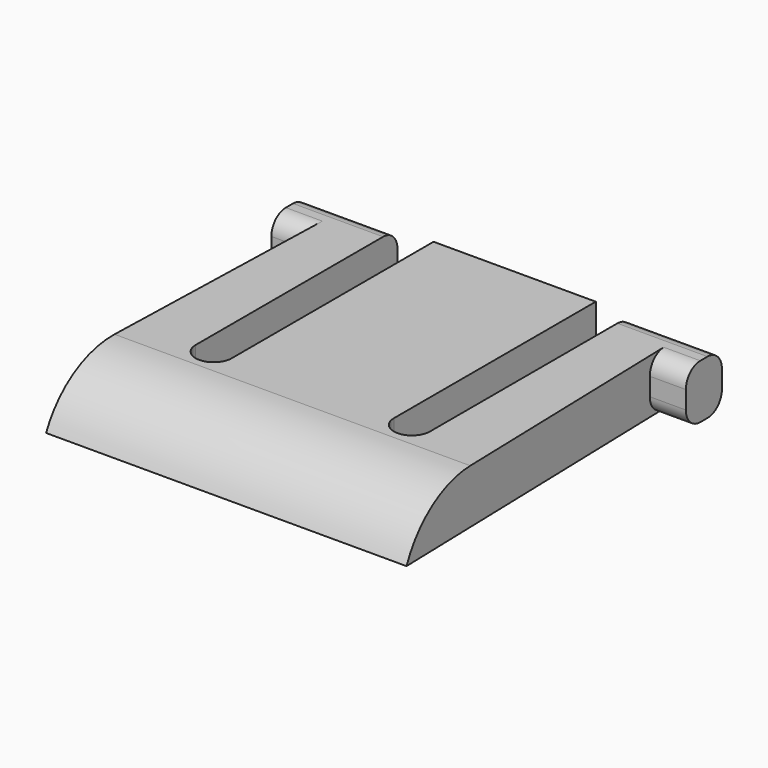
from build123d import *

# Parameters (mm, degrees)
F4_DEPTH    = 3
F1_R        = 1
F3_T1_DEPTH = 42.9128784748


# Not quite as in the source:
# - a fillet or chamfer that OpenCascade refuses, or shapes differently, is made with other operations: its cross-section is extruded or revolved along the edge and cut away or added


with BuildPart() as f4:
    # F0 (on Top) → F4 (new body)
    with BuildSketch(Plane.XY):
        with BuildLine():
            Line((0, 20), (0, 0))
            Line((0, 0), (10, 0))
            Line((10, 0), (9.5, 17.5))
            Line((9.5, 17.5), (11.5, 17.5))
            Line((11.5, 17.5), (11.5, 20))
            Line((11.5, 20), (6.5, 20))
            Line((6.5, 20), (6.5, 6))
            ThreePointArc((6.5, 6), (5.5, 5), (4.5, 6))
            Line((4.5, 6), (4.5, 20))
            Line((4.5, 20), (0, 20))
        make_face()
    extrude(amount=F4_DEPTH)

    # F1
    f1_edges = [f4.edges().sort_by_distance(p)[0] for p in [
        (10.5, 17.5, 3),
        (9, 20, 3),
        (10.5, 17.5, 0),
        (9, 20, 0),
    ]]
    fillet(f1_edges, radius=F1_R)

    # F2: F4 across plane


with BuildPart() as f4_1:
    add(f4.part)
    add(f4.part.mirror(Plane.YZ))

    # F3: fillet of radius 5 on 1 edges, made by hand

    # F3_s2 → F3_t1 (cut)
    with BuildSketch(Plane.YZ.offset(-21.4564392374)):
        with BuildLine():
            ThreePointArc((4.582575695, 3), (1.8439629074, 2.1833001327), (0, 0))
            Line((0, 0), (0, 3))
            Line((0, 3), (4.582575695, 3))
        make_face()
    extrude(amount=F3_T1_DEPTH, mode=Mode.SUBTRACT)


solid = f4_1.part
